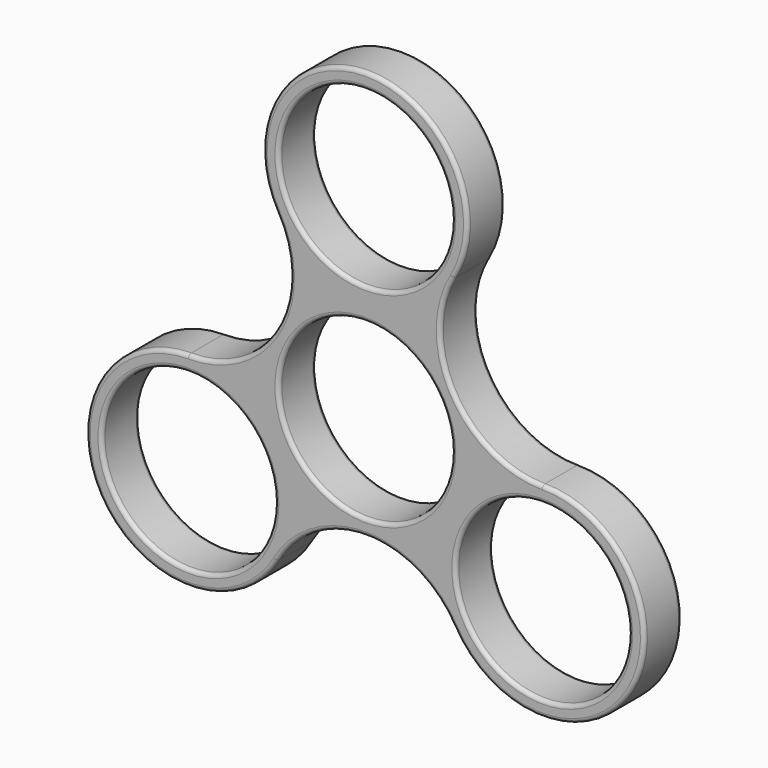
from build123d import *

# Parameters (mm, degrees)
F1_R     = 11.125
F2_DEPTH = 6
F3_R     = 0.5


# Not quite as in the source:
# - a feature names something its author has since deleted; it is built from what else it names


with BuildPart() as f2:
    # F1 (on Front) → F2 (new body)
    with BuildSketch(Plane.XZ):
        with BuildLine():
            ThreePointArc((-11.3665834247, 19.6875), (-11.3665834247, 6.5625), (-22.7331668493, 0))
            ThreePointArc((-22.7331668493, 0), (-34.099750274, -19.6875), (-11.3665834247, -19.6875))
            ThreePointArc((-11.3665834247, -19.6875), (0, -13.125), (11.3665834247, -19.6875))
            ThreePointArc((11.3665834247, -19.6875), (34.099750274, -19.6875), (22.7331668493, 0))
            ThreePointArc((22.7331668493, 0), (11.3665834247, 6.5625), (11.3665834247, 19.6875))
            ThreePointArc((11.3665834247, 19.6875), (0, 39.375), (-11.3665834247, 19.6875))
        make_face()
        with Locations((-22.7331668493, -13.125)):
            Circle(F1_R, mode=Mode.SUBTRACT)
        Circle(F1_R, mode=Mode.SUBTRACT)
        with Locations((22.7331668493, -13.125)):
            Circle(F1_R, mode=Mode.SUBTRACT)
        with Locations((0, 26.25)):
            Circle(F1_R, mode=Mode.SUBTRACT)
    extrude(amount=F2_DEPTH)

    # F3
    f3_edges = [f2.edges().sort_by_distance(p)[0] for p in [
        (11.366583, -6, 6.5625),
        (0, -6, 39.375),
        (-11.366583, -6, 6.5625),
        (-34.09975, -6, -19.6875),
        (0, -6, -13.125),
        (34.09975, -6, -19.6875),
        (-33.858167, -6, -13.125),
        (-11.125, -6, 0),
        (11.608167, -6, -13.125),
        (-11.125, -6, 26.25),
        (11.366583, 0, 6.5625),
        (0, 0, 39.375),
        (-11.366583, 0, 6.5625),
        (-34.09975, 0, -19.6875),
        (0, 0, -13.125),
        (34.09975, 0, -19.6875),
        (-33.858167, 0, -13.125),
        (-11.125, 0, 0),
        (11.608167, 0, -13.125),
        (-11.125, 0, 26.25),
    ]]
    fillet(f3_edges, radius=F3_R)


solid = f2.part
